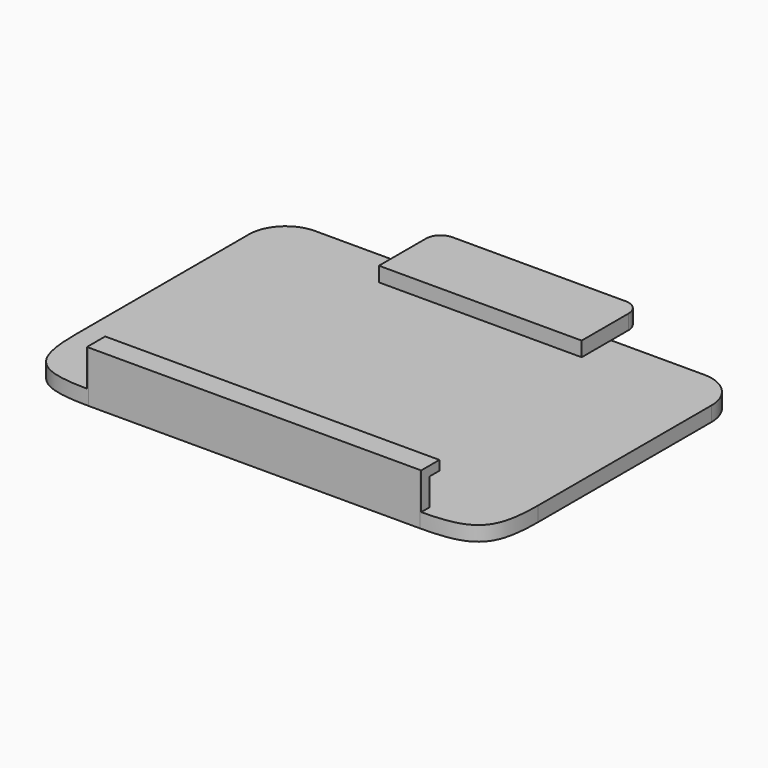
from build123d import *

# Parameters (mm, degrees)
F0_W        = 63
F0_H        = 43.5
F1_DEPTH    = 2
F2_R        = 5
F3_W        = 27.6
F3_H        = 5
F4_DEPTH    = 2
F5_R        = 2
F6_DEPTH    = 5
F7_W        = 45.5
F7_H        = 1.3
F8_DEPTH    = 1.7
F9_T1_DEPTH = 46.6629509039


# Not quite as in the source:
# - a fillet or chamfer that OpenCascade refuses, or shapes differently, is made with other operations: its cross-section is extruded or revolved along the edge and cut away or added


with BuildPart() as f1:
    # F0 (on Top) → F1 (new body)
    with BuildSketch(Plane.XY):
        with Locations((23.961127311, -16.9047259986)):
            Rectangle(F0_W, F0_H)
    extrude(amount=F1_DEPTH)

    # F2
    f2_edges = [f1.edges().sort_by_distance(p)[0] for p in [
        (-7.538873, 4.845274, 1),
        (55.461127, 4.845274, 1),
    ]]
    fillet(f2_edges, radius=F2_R)

    # F3 (on face) → F4 (join)
    with BuildSketch(Plane.XY.offset(2)):
        with Locations((23.961127311, 7.3452740014)):
            Rectangle(F3_W, F3_H)
        Polygon((10.161127311, -0.1547259986), (23.961127311, -0.1547259986), (37.761127311, -0.1547259986), (37.761127311, 4.8452740014), (10.161127311, 4.8452740014), align=None)
    extrude(amount=F4_DEPTH)

    # F5
    f5_edges = [f1.edges().sort_by_distance(p)[0] for p in [
        (10.161127, 9.845274, 3),
        (37.761127, 9.845274, 3),
    ]]
    fillet(f5_edges, radius=F5_R)

    # F3 (on face) → F6 (join)
    with BuildSketch(Plane.XY.offset(2)):
        Polygon((1.211127311, -37.2547259986), (1.211127311, -38.6547259986), (23.961127311, -38.6547259986), (46.711127311, -38.6547259986), (46.711127311, -37.2547259986), align=None)
    extrude(amount=F6_DEPTH)

    # F7 (on face) → F8 (join)
    with BuildSketch(Plane(origin=(0, -37.2547259986, 0), x_dir=(-1, 0, 0), z_dir=(0, 1, 0))):
        with Locations((-23.961127311, 6.35)):
            Rectangle(F7_W, F7_H)
    extrude(amount=F8_DEPTH)

    # F9: fillet of radius 8.9325901808 on 2 edges, made by hand

    # F9_s2 → F9_t1 (cut)
    with BuildSketch(Plane.XY.offset(-22.331475452)):
        with BuildLine():
            add(Edge.make_bspline(
                [(46.5285371302, -38.6547259986), (55.461127311, -38.6547259986), (55.461127311, -29.7221358179)],
                knots=[0, 0, 0, 1, 1, 1], degree=2, weights=[1, 1.5, 1]))
            Line((55.461127311, -29.7221358179), (55.461127311, -38.6547259986))
            Line((55.461127311, -38.6547259986), (46.5285371302, -38.6547259986))
        make_face()
        with BuildLine():
            add(Edge.make_bspline(
                [(-7.538872689, -29.7221358179), (-7.538872689, -38.6547259986), (1.3937174918, -38.6547259986)],
                knots=[0, 0, 0, 1, 1, 1], degree=2, weights=[1, 1.5, 1]))
            Line((1.3937174918, -38.6547259986), (-7.538872689, -38.6547259986))
            Line((-7.538872689, -38.6547259986), (-7.538872689, -29.7221358179))
        make_face()
    extrude(amount=F9_T1_DEPTH, mode=Mode.SUBTRACT)


solid = f1.part
